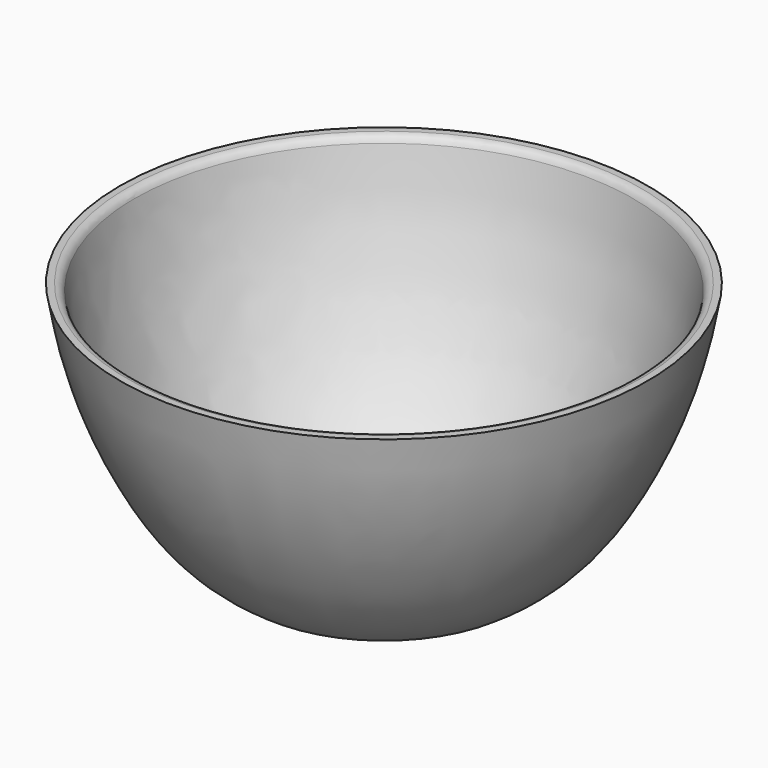
from build123d import *

# Parameters (mm, degrees)
F2_T = -2.5
F3_R = 1.5


with BuildPart() as f1:
    # F0 (on Front) → F1 (revolve)
    with BuildSketch(Plane.XZ):
        with BuildLine():
            Line((-25, 0), (0, 0))
            Line((0, 0), (0, 46.5909080625))
            Line((0, 46.5909080625), (-50, 46.5909080625))
            add(Edge.make_bspline(
                [(-25, 0), (-32.0024192333, 4.4779088348), (-41.2479135414, 16.8069449168), (-47.999671412, 34.1533497409), (-50, 46.5909080625)],
                knots=[0, 0, 0, 0, 0.458566155, 1, 1, 1, 1], degree=3))
        make_face()
    revolve(axis=Axis((0, 0, 23.2954540313), (0, 0, 1)))

    # F2
    f2_openings = [f1.faces().sort_by_distance(p)[0] for p in [
        (0, 0, 46.590908),
    ]]
    offset(amount=F2_T, openings=f2_openings)

    # F3
    f3_edges = [f1.edges().sort_by_distance(p)[0] for p in [
        (47.467126, 0, 46.590908),
    ]]
    fillet(f3_edges, radius=F3_R)


solid = f1.part
